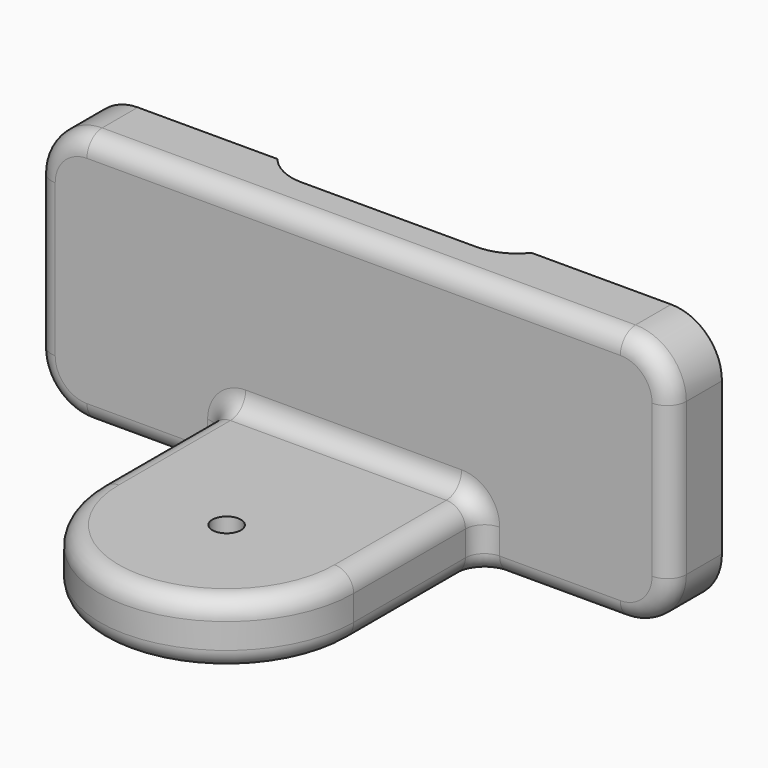
from build123d import *

# Parameters (mm, degrees)
F0_W          = 100
F0_H          = 40
F1_DEPTH      = 10
F3_DEPTH      = 10
F4_W          = 40
F4_H          = 3
F5_DEPTH      = 40.001
F6_R          = 2.25
F7_DEPTH      = 40.001
F8_R          = 4.5
F9_DEPTH      = 5.7
F10_T1_DEPTH  = 40
F10_T3_DEPTH  = 40
F10_T5_DEPTH  = 50
F10_T7_DEPTH  = 50
F10_T9_DEPTH  = 50
F10_T11_DEPTH = 50
F11_F1_R      = 3
F11_F2_R      = 3
F11_F3_R      = 3


# Not quite as in the source:
# - a fillet or chamfer that OpenCascade refuses, or shapes differently, is made with other operations: its cross-section is extruded or revolved along the edge and cut away or added


with BuildPart() as f1:
    # F0 (on Front) → F1 (new body)
    with BuildSketch(Plane.XZ):
        with Locations((50, 20)):
            Rectangle(F0_W, F0_H)
    extrude(amount=F1_DEPTH)

    # F2 (on Top) → F3 (join)
    with BuildSketch(Plane.XY):
        with BuildLine():
            Line((70, 0), (30, 0))
            Line((30, 0), (30, -35))
            ThreePointArc((30, -35), (50, -55), (70, -35))
            Line((70, -35), (70, 0))
        make_face()
    extrude(amount=F3_DEPTH)

    # F4 (on face) → F5 (cut, through all)
    with BuildSketch(Plane(origin=(0, 0, 0), x_dir=(1, 0, 0), z_dir=(0, 0, -1))):
        with Locations((50, 1.5)):
            Rectangle(F4_W, F4_H)
    extrude(amount=-F5_DEPTH, mode=Mode.SUBTRACT)

    # F6 (on face) → F7 (cut, through all)
    with BuildSketch(Plane(origin=(0, 0, 0), x_dir=(1, 0, 0), z_dir=(0, 0, -1))):
        with Locations((50, 35)):
            Circle(F6_R)
    extrude(amount=-F7_DEPTH, mode=Mode.SUBTRACT)

    # F8 (on face) → F9 (cut)
    with BuildSketch(Plane(origin=(0, 0, 0), x_dir=(1, 0, 0), z_dir=(0, 0, -1))):
        with Locations((50, 35)):
            Circle(F8_R)
    extrude(amount=-F9_DEPTH, mode=Mode.SUBTRACT)

    # F10: fillet of radius 8 on 6 edges, made by hand

    # F10_s2 → F10_t1 (join)
    with BuildSketch(Plane.XY):
        with BuildLine():
            ThreePointArc((70, 0), (67.2191036167, -2.2111025509), (63.7550020016, -3))
            Line((63.7550020016, -3), (70, -3))
            Line((70, -3), (70, 0))
        make_face()
    extrude(amount=F10_T1_DEPTH)

    # F10_s4 → F10_t3 (join)
    with BuildSketch(Plane.XY):
        with BuildLine():
            ThreePointArc((36.2449979984, -3), (32.7808963833, -2.2111025509), (30, 0))
            Line((30, 0), (30, -3))
            Line((30, -3), (36.2449979984, -3))
        make_face()
    extrude(amount=F10_T3_DEPTH)

    # F10_s6 → F10_t5 (cut)
    with BuildSketch(Plane.XZ.offset(-20)):
        with BuildLine():
            ThreePointArc((0, 32), (2.3431457505, 37.6568542495), (8, 40))
            Line((8, 40), (0, 40))
            Line((0, 40), (0, 32))
        make_face()
    extrude(amount=F10_T5_DEPTH, mode=Mode.SUBTRACT)

    # F10_s8 → F10_t7 (cut)
    with BuildSketch(Plane.XZ.offset(-20)):
        with BuildLine():
            ThreePointArc((0, 8), (2.3431457505, 2.3431457505), (8, 0))
            Line((8, 0), (0, 0))
            Line((0, 0), (0, 8))
        make_face()
    extrude(amount=F10_T7_DEPTH, mode=Mode.SUBTRACT)

    # F10_s10 → F10_t9 (cut)
    with BuildSketch(Plane.XZ.offset(-20)):
        with BuildLine():
            ThreePointArc((92, 40), (97.6568542495, 37.6568542495), (100, 32))
            Line((100, 32), (100, 40))
            Line((100, 40), (92, 40))
        make_face()
    extrude(amount=F10_T9_DEPTH, mode=Mode.SUBTRACT)

    # F10_s12 → F10_t11 (cut)
    with BuildSketch(Plane.XZ.offset(-20)):
        with BuildLine():
            ThreePointArc((92, 0), (97.6568542495, 2.3431457505), (100, 8))
            Line((100, 8), (100, 0))
            Line((100, 0), (92, 0))
        make_face()
    extrude(amount=F10_T11_DEPTH, mode=Mode.SUBTRACT)

    # F11: fillet of radius 3 on 17 edges, made by hand

    # F11_f1
    f11_f1_edges = [f1.edges().sort_by_distance(p)[0] for p in [
        (50, -55, 10),
        (70, -22.5, 10),
        (30, -22.5, 10),
    ]]
    fillet(f11_f1_edges, radius=F11_F1_R)

    # F11_f2
    f11_f2_edges = [f1.edges().sort_by_distance(p)[0] for p in [
        (70, -10, 3.5),
        (50, -10, 10),
        (69.1213203436, -10, 9.1213203436),
        (30.8786796564, -10, 9.1213203436),
    ]]
    fillet(f11_f2_edges, radius=F11_F2_R)

    # F11_f3
    f11_f3_edges = [f1.edges().sort_by_distance(p)[0] for p in [
        (50, -55, 0),
        (0, -10, 20),
        (2.3431457505, -10, 2.3431457505),
        (17.5, -10, 0),
        (2.3431457505, -10, 37.6568542495),
        (50, -10, 40),
        (97.6568542495, -10, 37.6568542495),
        (100, -10, 20),
        (97.6568542495, -10, 2.3431457505),
        (82.5, -10, 0),
        (70, -24, 0),
        (30, -24, 0),
        (29.1213203436, -10.8786796564, 0),
        (70.8786796564, -10.8786796564, 0),
    ]]
    fillet(f11_f3_edges, radius=F11_F3_R)


solid = f1.part
